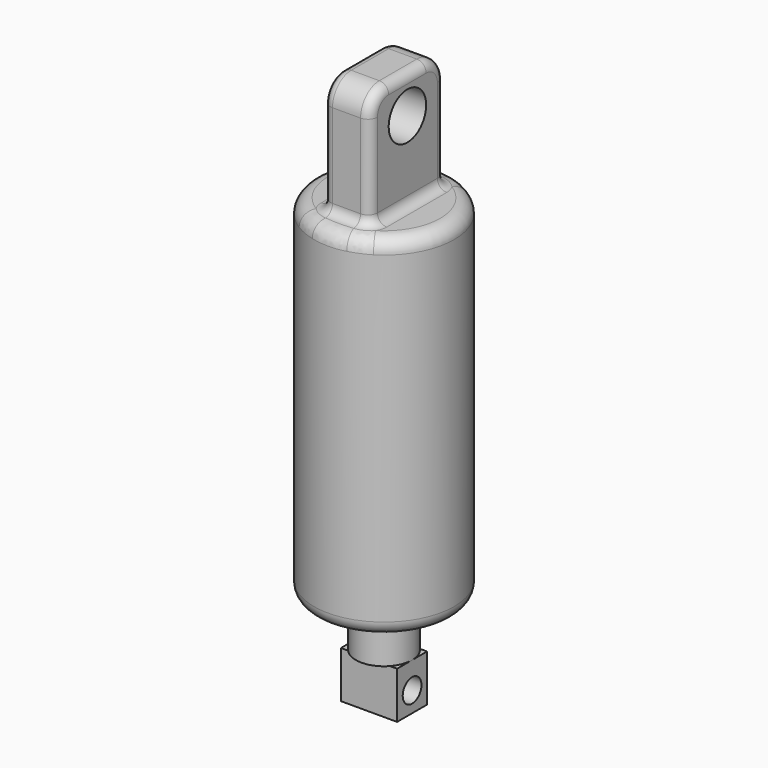
from build123d import *

# Parameters (mm, degrees)
F0_R      = 15
F1_DEPTH  = 70
F2_R      = 14
F3_DEPTH  = 65
F4_R      = 15
F4_R_2    = 14
F4_R_3    = 6
F5_DEPTH  = 5
F6_W      = 10
F6_H      = 20
F7_DEPTH  = 25
F8_R      = 5
F9_DEPTH  = 25
F10_R     = 5
F11_R     = 2
F12_R     = 14
F13_DEPTH = 5
F14_R     = 6
F15_DEPTH = 75
F17_DEPTH = 10
F18_R     = 2.5
F19_DEPTH = 25
F20_R     = 3


with BuildPart() as f1:
    # F0 (on Top) → F1 (new body)
    with BuildSketch(Plane.XY):
        Circle(F0_R)
    extrude(amount=F1_DEPTH)

    # F2 (on face) → F3 (cut)
    with BuildSketch(Plane(origin=(0, 0, 0), x_dir=(1, 0, 0), z_dir=(0, 0, -1))):
        with Locations((-0.4053307348, 0)):
            Circle(F2_R)
    extrude(amount=-F3_DEPTH, mode=Mode.SUBTRACT)

    # F4 (on face) → F5 (join)
    with BuildSketch(Plane(origin=(0, 0, 0), x_dir=(1, 0, 0), z_dir=(0, 0, -1))):
        Circle(F4_R)
        with Locations((-0.4053307348, 0)):
            Circle(F4_R_2, mode=Mode.SUBTRACT)
        with Locations((-0.4053307348, 0)):
            Circle(F4_R_2)
        Circle(F4_R_3, mode=Mode.SUBTRACT)
    extrude(amount=F5_DEPTH)

    # F6 (on face) → F7 (join)
    with BuildSketch(Plane.XY.offset(70)):
        Rectangle(F6_W, F6_H)
    extrude(amount=F7_DEPTH)

    # F8 (on face) → F9 (cut)
    with BuildSketch(Plane(origin=(-5, 0, 0), x_dir=(0, -1, 0), z_dir=(-1, 0, 0))):
        with Locations((0, 87)):
            Circle(F8_R)
    extrude(amount=-F9_DEPTH, mode=Mode.SUBTRACT)

    # F10
    f10_edges = [f1.edges().sort_by_distance(p)[0] for p in [
        (0, 10, 95),
        (0, -10, 95),
    ]]
    fillet(f10_edges, radius=F10_R)

    # F11
    f11_edges = [f1.edges().sort_by_distance(p)[0] for p in [
        (-5, 10, 80),
        (5, 10, 80),
        (5, 0, 70),
        (5, -10, 80),
        (5, -8.535534, 93.535534),
        (5, 0, 95),
        (5, 8.535534, 93.535534),
        (-5, -10, 80),
        (0, -10, 70),
        (-5, -8.535534, 93.535534),
        (0, 10, 70),
        (-5, 0, 70),
        (-5, 0, 95),
        (-5, 8.535534, 93.535534),
    ]]
    fillet(f11_edges, radius=F11_R)

    # F20
    f20_edges = [f1.edges().sort_by_distance(p)[0] for p in [
        (-15, 0, -5),
        (-15, 0, 70),
    ]]
    fillet(f20_edges, radius=F20_R)


with BuildPart() as f13:
    # F12 (on face) → F13 (new body)
    with BuildSketch(Plane(origin=(0, 0, 65), x_dir=(1, 0, 0), z_dir=(0, 0, -1))):
        Circle(F12_R)
    extrude(amount=F13_DEPTH)

    # F14 (on face) → F15 (join)
    with BuildSketch(Plane(origin=(0, 0, 60), x_dir=(1, 0, 0), z_dir=(0, 0, -1))):
        Circle(F14_R)
    extrude(amount=F15_DEPTH)

    # F16 (on face) → F17 (join)
    with BuildSketch(Plane(origin=(0, 0, -15), x_dir=(1, 0, 0), z_dir=(0, 0, -1))):
        with BuildLine():
            Line((6, 0), (6, 4))
            Line((6, 4), (4.472135955, 4))
            ThreePointArc((4.472135955, 4), (5.6050341538, 2.1409325386), (6, 0))
        make_face()
        with BuildLine():
            ThreePointArc((6, 0), (5.6050341538, 2.1409325386), (4.472135955, 4))
            Line((4.472135955, 4), (-4.472135955, 4))
            ThreePointArc((-4.472135955, 4), (-5.6050341538, 2.1409325386), (-6, 0))
            ThreePointArc((-6, 0), (-5.6050341538, -2.1409325386), (-4.472135955, -4))
            Line((-4.472135955, -4), (4.472135955, -4))
            ThreePointArc((4.472135955, -4), (5.6050341538, -2.1409325386), (6, 0))
        make_face()
        with BuildLine():
            ThreePointArc((-6, 0), (-5.6050341538, 2.1409325386), (-4.472135955, 4))
            Line((-4.472135955, 4), (-6, 4))
            Line((-6, 4), (-6, 0))
        make_face()
        with BuildLine():
            ThreePointArc((-4.472135955, -4), (-5.6050341538, -2.1409325386), (-6, 0))
            Line((-6, 0), (-6, -4))
            Line((-6, -4), (-4.472135955, -4))
        make_face()
        with BuildLine():
            Line((6, -4), (6, 0))
            ThreePointArc((6, 0), (5.6050341538, -2.1409325386), (4.472135955, -4))
            Line((4.472135955, -4), (6, -4))
        make_face()
    extrude(amount=F17_DEPTH)

    # F18 (on face) → F19 (cut)
    with BuildSketch(Plane.YZ.offset(6)):
        with Locations((0, -20.694527775)):
            Circle(F18_R)
    extrude(amount=-F19_DEPTH, mode=Mode.SUBTRACT)


solid = Compound([f1.part, f13.part])
